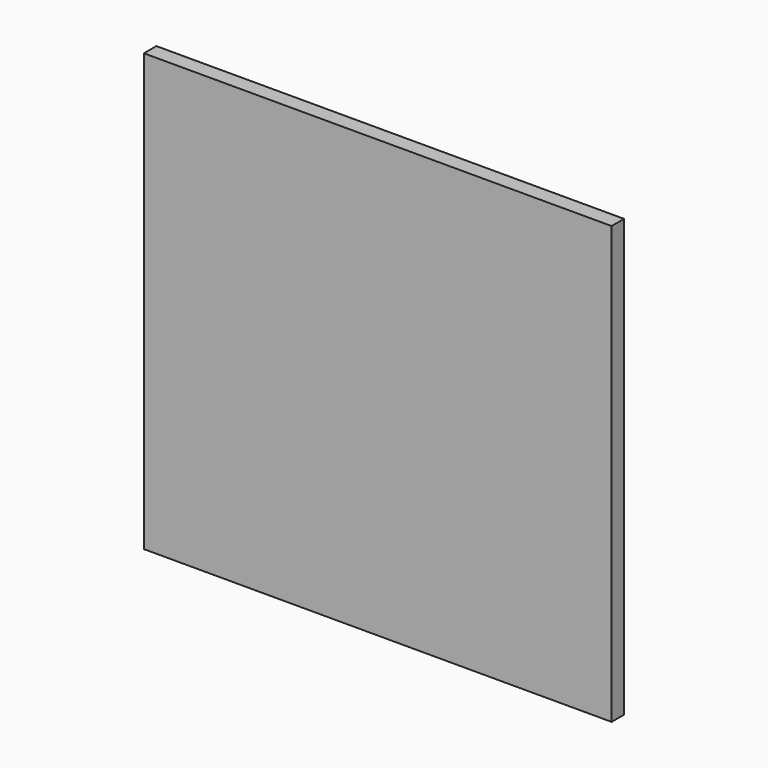
from build123d import *

# Parameters (mm, degrees)
F0_W     = 381
F0_H     = 355.6
F2_DEPTH = 12.7


# Not quite as in the source:
# - a variable given as a bare number and used for a length is read in inches; the dataset says mm whatever the document's units were


with BuildPart() as f2:
    # F0 (on Front) → F2 (new body)
    with BuildSketch(Plane.XZ):
        with Locations((190.5, -177.8)):
            Rectangle(F0_W, F0_H)
    extrude(amount=F2_DEPTH)


solid = f2.part
